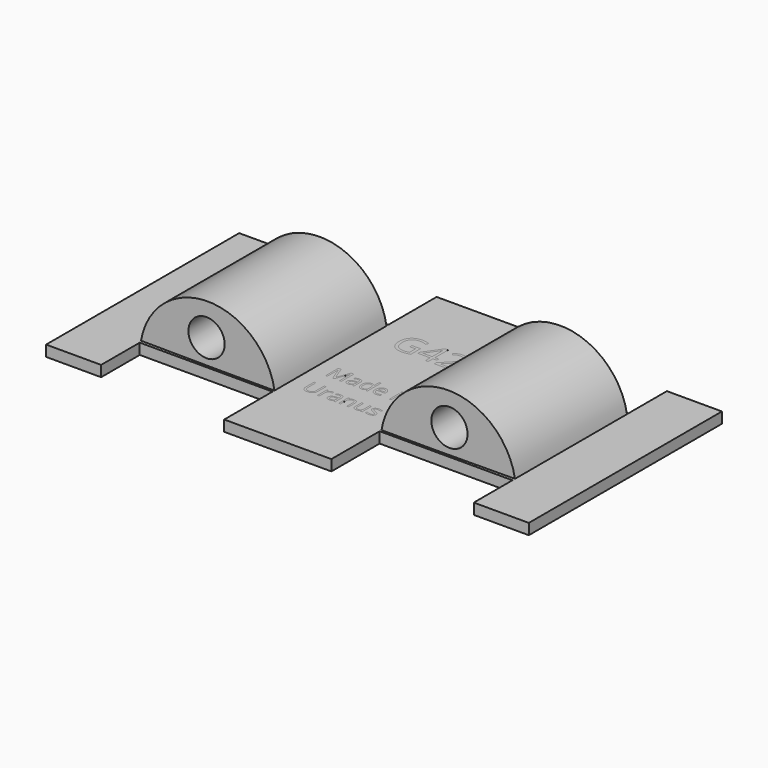
from build123d import *

# Parameters (mm, degrees)
F1_DEPTH       = 2.286
F2_R           = 3.8106547992
F3_DEPTH       = 14.732
F4_TEXT_SIZE   = 7.3900866684
F4_TEXT_SIZE_2 = 4.6530175799
F5_DEPTH       = 0.000254
F6_W           = 22.5534540367
F6_H           = 2.286
F7_DEPTH       = 2.54
F8_W           = 22.5534540367
F8_H           = 2.286
F9_DEPTH       = 2.54


# Not quite as in the source:
# - Text() gives the source's letters only with a copy of the font that has no kerning and outlines rounded to 1/6400 em; it was checked with that copy


with BuildPart() as f1:
    # F0 (on Top) → F1 (new body)
    with BuildSketch(Plane.XY):
        Polygon((39.2167270184, -25.4), (50.8, -25.4), (50.8, 25.4), (39.2167270184, 25.4), (39.2167270184, 15.24), (11.2767270184, 15.24), (11.2767270184, 25.4), (-11.2767270184, 25.4), (-11.2767270184, 15.24), (-39.2167270184, 15.24), (-39.2167270184, 25.4), (-50.8, 25.4), (-50.8, -25.4), (-39.2167270184, -25.4), (-39.2167270184, -15.24), (-11.2767270184, -15.24), (-11.2767270184, -25.4), (11.2767270184, -25.4), (11.2767270184, -15.24), (39.2167270184, -15.24), align=None)
    extrude(amount=F1_DEPTH)

    # F2 (on Front) → F3 (join, symmetric)
    with BuildSketch(Plane.XZ):
        with BuildLine():
            Line((-39.3549734488, 2.3931630209), (-11.2439553667, 2.2112238898))
            ThreePointArc((-11.2439553667, 2.2112238898), (-25.2221828213, 14.2428027126), (-39.3549734488, 2.3931630209))
        make_face()
        with Locations((-25.5629364401, 7.4394908734)):
            Circle(F2_R, mode=Mode.SUBTRACT)
        with BuildLine():
            ThreePointArc((39.3549734488, 2.3931630209), (25.2221828213, 14.2428027126), (11.2439553667, 2.2112238898))
            Line((11.2439553667, 2.2112238898), (39.3549734488, 2.3931630209))
        make_face()
        with Locations((25.5629364401, 7.4394908734)):
            Circle(F2_R, mode=Mode.SUBTRACT)
    extrude(amount=F3_DEPTH, both=True)

    # F4 (on face) → F5 (join)
    with BuildSketch(Plane.XY.offset(2.286)):
        with Locations((-6.6644959152, 9.1276527382)):
            Text('G42', F4_TEXT_SIZE, font='Open Sans', text_align=(TextAlign.LEFT, TextAlign.BOTTOM))
        with Locations((-8.473965805, -5.3208624013)):
            Text('Made in', F4_TEXT_SIZE_2, font='Open Sans', text_align=(TextAlign.LEFT, TextAlign.BOTTOM))
        with Locations((-8.473965805, -11.6489663099)):
            Text('Uranus', F4_TEXT_SIZE_2, font='Open Sans', text_align=(TextAlign.LEFT, TextAlign.BOTTOM))
    extrude(amount=F5_DEPTH)

    # F6 (on face) → F7 (join)
    with BuildSketch(Plane(origin=(0, 25.4, 0), x_dir=(-1, 0, 0), z_dir=(0, 1, 0))):
        with Locations((0, 1.143)):
            Rectangle(F6_W, F6_H)
    extrude(amount=F7_DEPTH)

    # F8 (on face) → F9 (join)
    with BuildSketch(Plane.XZ.offset(25.4)):
        with Locations((0, 1.143)):
            Rectangle(F8_W, F8_H)
    extrude(amount=F9_DEPTH)


solid = f1.part
